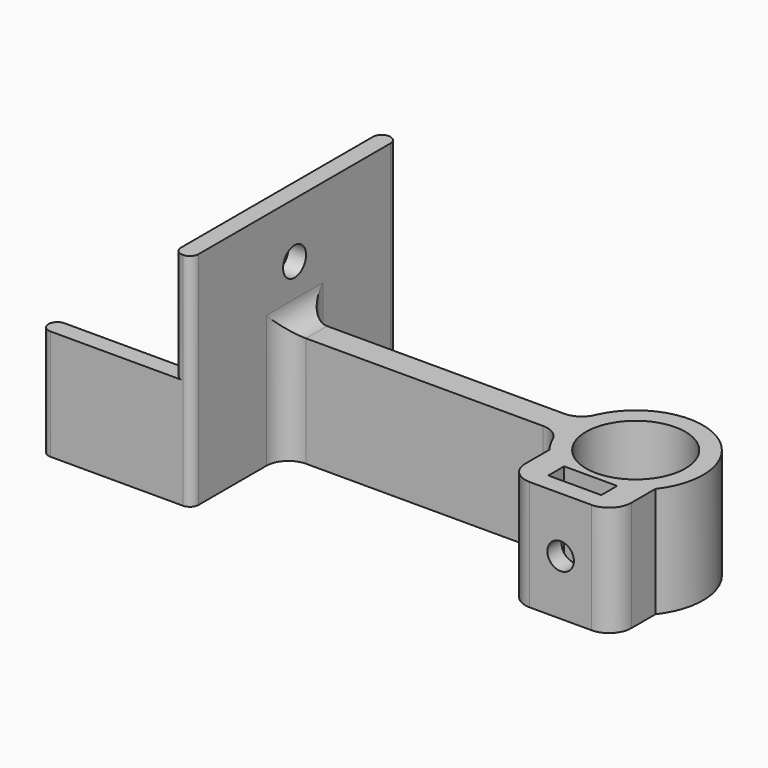
from build123d import *

# Parameters (mm, degrees)
F0_R     = 11.25
F1_DEPTH = 25
F3_DEPTH = 25
F4_R     = 3.25
F5_DEPTH = 4
F6_W     = 12
F6_H     = 4.5
F7_DEPTH = 19
F8_R     = 3
F9_DEPTH = 12
F10_R    = 5
F11_R    = 5
F12_R    = 1.99999


# Not quite as in the source:
# - a fillet or chamfer is up to 0.001 mm smaller than in the source, because OpenCascade refuses the exact size


with BuildPart() as f1:
    # F0 (on Top) → F1 (new body)
    with BuildSketch(Plane.XY):
        with BuildLine():
            Line((-81.25, 25.15), (-81.25, -25.15))
            Line((-81.25, -25.15), (-111.25, -25.15))
            Line((-111.25, -25.15), (-111.25, -29.15))
            Line((-111.25, -29.15), (-77.25, -29.15))
            Line((-77.25, -29.15), (-77.25, -3))
            Line((-77.25, -3), (-14.9520065543, -3))
            ThreePointArc((-14.9520065543, -3), (-13.8519724825, -6.3785075325), (-12, -9.4107651124))
            Line((-12, -9.4107651124), (-12, -12.3110722522))
            Line((-12, -12.3110722522), (-12, -21.25))
            Line((-12, -21.25), (-9, -21.25))
            Line((-9, -21.25), (9, -21.25))
            Line((9, -21.25), (12, -21.25))
            Line((12, -21.25), (12, -12.3110722522))
            Line((12, -12.3110722522), (12, -9.4107651124))
            ThreePointArc((12, -9.4107651124), (6.3785075325, 13.8519724825), (-14.9520065543, 3))
            Line((-14.9520065543, 3), (-77.25, 3))
            Line((-77.25, 3), (-77.25, 29.15))
            Line((-77.25, 29.15), (-111.25, 29.15))
            Line((-111.25, 29.15), (-111.25, 25.15))
            Line((-111.25, 25.15), (-81.25, 25.15))
        make_face()
        Circle(F0_R, mode=Mode.SUBTRACT)
    extrude(amount=F1_DEPTH)

    # F2 (on face) → F3 (join)
    with BuildSketch(Plane.XY.offset(25)):
        Polygon((-77.25, 3), (-77.25, 29.15), (-81.25, 29.15), (-81.25, 25.15), (-81.25, -25.15), (-81.25, -29.15), (-77.25, -29.15), (-77.25, -3), align=None)
    extrude(amount=F3_DEPTH)

    # F4 (on face) → F5 (cut)
    with BuildSketch(Plane.YZ.offset(-77.25)):
        with Locations((0, 37.5)):
            Circle(F4_R)
    extrude(amount=-F5_DEPTH, mode=Mode.SUBTRACT)

    # F6 (on face) → F7 (cut)
    with BuildSketch(Plane.XY.offset(25)):
        with Locations((0, -15)):
            Rectangle(F6_W, F6_H)
    extrude(amount=-F7_DEPTH, mode=Mode.SUBTRACT)

    # F8 (on face) → F9 (cut)
    with BuildSketch(Plane.XZ.offset(21.25)):
        with Locations((0, 12.5)):
            Circle(F8_R)
    extrude(amount=-F9_DEPTH, mode=Mode.SUBTRACT)

    # F10
    f10_edges = [f1.edges().sort_by_distance(p)[0] for p in [
        (12, -21.25, 12.5),
        (-12, -21.25, 12.5),
        (-77.25, -3, 12.5),
        (-77.25, 3, 12.5),
    ]]
    fillet(f10_edges, radius=F10_R)

    # F11
    f11_edges = [f1.edges().sort_by_distance(p)[0] for p in [
        (-14.952007, 3, 12.5),
        (-14.952007, -3, 12.5),
        (-77.25, 0, 25),
    ]]
    fillet(f11_edges, radius=F11_R)

    # F12 (radius 2 in the source; OpenCascade refuses exactly that, so slightly less here)
    f12_edges = [f1.edges().sort_by_distance(p)[0] for p in [
        (-111.25, 29.15, 12.5),
        (-111.25, -25.15, 12.5),
        (-111.25, -29.15, 12.5),
        (-111.25, 25.15, 12.5),
        (-77.25, 29.15, 25),
        (-81.25, 29.15, 37.5),
        (-77.25, -29.15, 25),
        (-81.25, -29.15, 37.5),
    ]]
    fillet(f12_edges, radius=F12_R)


solid = f1.part
